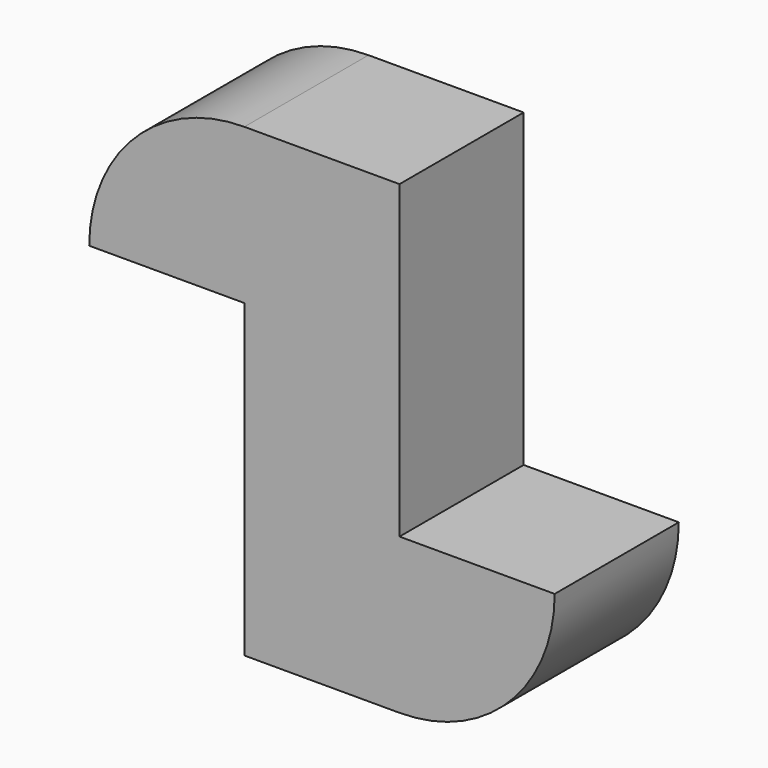
from build123d import *

# Parameters (mm, degrees)
F0_W     = 50.8
F0_H     = 25.4
F1_DEPTH = 25.4
F2_W     = 25.4
F2_H     = 25.4
F3_DEPTH = 50.8
F4_W     = 25.4
F4_H     = 25.4
F5_DEPTH = 25.4
F6_R     = 25.39999


# Not quite as in the source:
# - a fillet or chamfer is up to 0.001 mm smaller than in the source, because OpenCascade refuses the exact size


with BuildPart() as f1:
    # F0 (on Top) → F1 (new body)
    with BuildSketch(Plane.XY):
        with Locations((25.4, 12.7)):
            Rectangle(F0_W, F0_H)
    extrude(amount=F1_DEPTH)

    # F2 (on face) → F3 (join)
    with BuildSketch(Plane.XY.offset(25.4)):
        with Locations((12.7, 12.7)):
            Rectangle(F2_W, F2_H)
    extrude(amount=F3_DEPTH)

    # F4 (on face) → F5 (join)
    with BuildSketch(Plane(origin=(0, 0, 0), x_dir=(0, -1, 0), z_dir=(-1, 0, 0))):
        with Locations((-12.7, 63.5)):
            Rectangle(F4_W, F4_H)
    extrude(amount=F5_DEPTH)

    # F6 (radius 25.4 in the source; OpenCascade refuses exactly that, so slightly less here)
    f6_edges = [f1.edges().sort_by_distance(p)[0] for p in [
        (50.8, 12.7, 0),
        (-25.4, 12.7, 76.2),
    ]]
    fillet(f6_edges, radius=F6_R)


solid = f1.part
